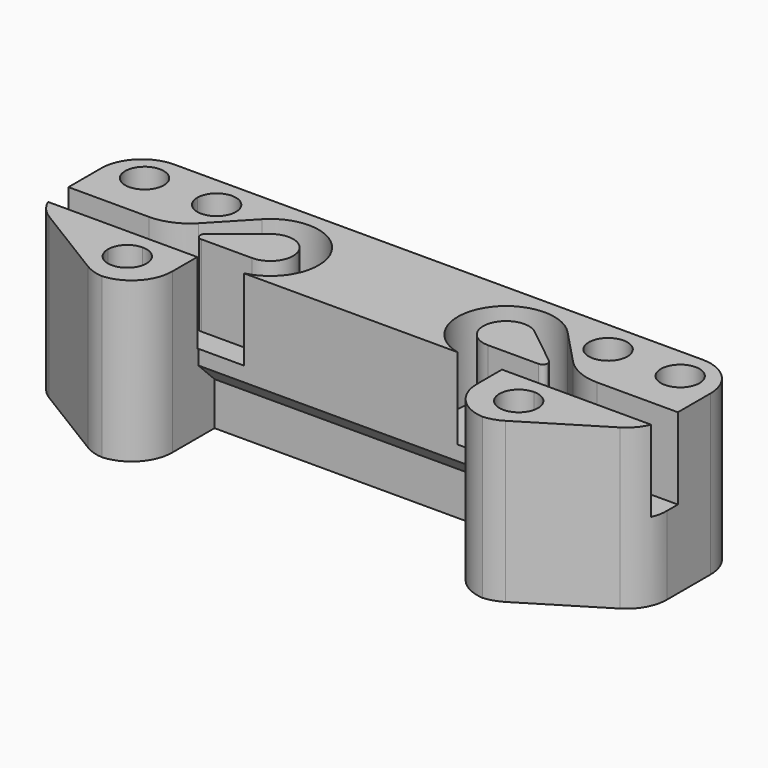
from build123d import *

# Parameters (mm, degrees)
F1_DEPTH    = 15.7
F2_W        = 10.0960650777
F2_H        = 2.9
F3_DEPTH    = 8
F4_R        = 5
F5_T1_DEPTH = 26.8923143391
F5_T3_DEPTH = 21.3473434867
F5_T5_DEPTH = 35.7
F6_W        = 15
F6_H        = 6.25
F7_DEPTH    = 2
F8_SIZE     = 1.99999


# Not quite as in the source:
# - a fillet or chamfer that OpenCascade refuses, or shapes differently, is made with other operations: its cross-section is extruded or revolved along the edge and cut away or added
# - a fillet or chamfer is up to 0.001 mm smaller than in the source, because OpenCascade refuses the exact size


with BuildPart() as f1:
    # F0 (on Top) → F1 (new body)
    with BuildSketch(Plane.XY):
        Polygon((30, 9), (0, 9), (0, -1.8), (15, -1.8), (15, -9), (19.5954625243, -9), (30, -2.6151265483), align=None)
        with BuildLine():
            ThreePointArc((21.17, -5.2), (17.9264971157, -6.5435028843), (19.27, -3.3))
            ThreePointArc((19.27, -3.3), (20.6135028843, -3.8564971157), (21.17, -5.2))
        make_face(mode=Mode.SUBTRACT)
        with BuildLine():
            ThreePointArc((19.27, 3.9), (17.9264971157, 7.1435028843), (21.17, 5.8))
            ThreePointArc((21.17, 5.8), (20.6135028843, 4.4564971157), (19.27, 3.9))
        make_face(mode=Mode.SUBTRACT)
        with BuildLine():
            ThreePointArc((24.47, 5.8), (26.37, 7.7), (28.27, 5.8))
            ThreePointArc((28.27, 5.8), (26.37, 3.9), (24.47, 5.8))
        make_face(mode=Mode.SUBTRACT)
    extrude(amount=F1_DEPTH)

    # F2 (on face) → F3 (cut)
    with BuildSketch(Plane.XY.offset(15.7)):
        with BuildLine():
            ThreePointArc((11.6039349223, 0.5750306588), (9.4802536205, 3.5683191144), (13.0070529624, 4.5839393448))
            Line((13.0070529624, 4.5839393448), (16.2772942688, 1.9751998411))
            ThreePointArc((16.2772942688, 1.9751998411), (16.3347359589, 2.3983908199), (16.3539349223, 2.8250306588))
            ThreePointArc((16.3539349223, 2.8250306588), (16.0161356009, 4.5842876531), (15.050783271, 6.09332325))
            ThreePointArc((15.050783271, 6.09332325), (7.4840088208, 5.1890756918), (10.5215341623, -1.8))
            Line((10.5215341623, -1.8), (12.6863356823, -1.8))
            ThreePointArc((12.6863356823, -1.8), (14.4922032842, -0.9459646832), (15.787235055, 0.5750306588))
            Line((15.787235055, 0.5750306588), (11.6039349223, 0.5750306588))
        make_face()
        with BuildLine():
            ThreePointArc((16.3539349223, 2.8250306588), (16.3347359589, 2.3983908199), (16.2772942688, 1.9751998411))
            Line((16.2772942688, 1.9751998411), (16.9157389312, 1.4658992557))
            ThreePointArc((16.9157389312, 1.4658992557), (17.0544357572, 1.2919384682), (17.1039349223, 1.0750306588))
            ThreePointArc((17.1039349223, 1.0750306588), (16.9574883129, 0.7214772682), (16.6039349223, 0.5750306588))
            Line((16.6039349223, 0.5750306588), (15.787235055, 0.5750306588))
            ThreePointArc((15.787235055, 0.5750306588), (14.4922032842, -0.9459646832), (12.6863356823, -1.8))
            Line((12.6863356823, -1.8), (15, -1.8))
            Line((15, -1.8), (15, -1.9249693412))
            Line((15, -1.9249693412), (19.9039349223, -1.9249693412))
            Line((19.9039349223, -1.9249693412), (19.9039349223, 0.9750306588))
            Line((19.9039349223, 0.9750306588), (15.050783271, 6.09332325))
            ThreePointArc((15.050783271, 6.09332325), (16.0161356009, 4.5842876531), (16.3539349223, 2.8250306588))
        make_face()
        with Locations((24.9519674612, -0.4749693412)):
            Rectangle(F2_W, F2_H)
    extrude(amount=-F3_DEPTH, mode=Mode.SUBTRACT)

    # F4
    f4_edges = [f1.edges().sort_by_distance(p)[0] for p in [
        (19.903935, 0.975031, 11.7),
    ]]
    fillet(f4_edges, radius=F4_R)

    # F5: fillet of radius 4 on 4 edges, made by hand

    # F5_s2 → F5_t1 (cut)
    with BuildSketch(Plane.XY.offset(-5.5961571696)):
        with BuildLine():
            ThreePointArc((30, -0.3766636805), (29.4905957559, -2.3300559271), (28.0921293656, -3.7859150232))
            Line((28.0921293656, -3.7859150232), (30, -2.6151265483))
            Line((30, -2.6151265483), (30, -0.3766636805))
        make_face()
    extrude(amount=F5_T1_DEPTH, mode=Mode.SUBTRACT)

    # F5_s4 → F5_t3 (cut)
    with BuildSketch(Plane.XY.offset(-2.8236717433)):
        with BuildLine():
            ThreePointArc((20.5581231925, -8.4092513427), (19.5529608525, -8.8494808332), (18.465993827, -9))
            Line((18.465993827, -9), (19.5954625243, -9))
            Line((19.5954625243, -9), (20.5581231925, -8.4092513427))
        make_face()
    extrude(amount=F5_T3_DEPTH, mode=Mode.SUBTRACT)

    # F5_s6 → F5_t5 (cut)
    with BuildSketch(Plane.XY.offset(-10)):
        with BuildLine():
            ThreePointArc((15, -5), (16.1715728753, -7.8284271247), (19, -9))
            Line((19, -9), (15, -9))
            Line((15, -9), (15, -5))
        make_face()
        with BuildLine():
            ThreePointArc((30, 5), (28.8284271247, 7.8284271247), (26, 9))
            Line((26, 9), (30, 9))
            Line((30, 9), (30, 5))
        make_face()
    extrude(amount=F5_T5_DEPTH, mode=Mode.SUBTRACT)

    # F6 (on face) → F7 (cut)
    with BuildSketch(Plane.XZ.offset(1.8)):
        with Locations((7.5, 3.125)):
            Rectangle(F6_W, F6_H)
    extrude(amount=-F7_DEPTH, mode=Mode.SUBTRACT)

    # F8 (size 2 in the source; OpenCascade refuses exactly that, so slightly less here)
    f8_edges = [f1.edges().sort_by_distance(p)[0] for p in [
        (7.5, 0.2, 6.25),
    ]]
    chamfer(f8_edges, length=F8_SIZE)

    # F9: F1 across plane


with BuildPart() as f1_1:
    add(f1.part)
    add(f1.part.mirror(Plane.YZ))


solid = f1_1.part
